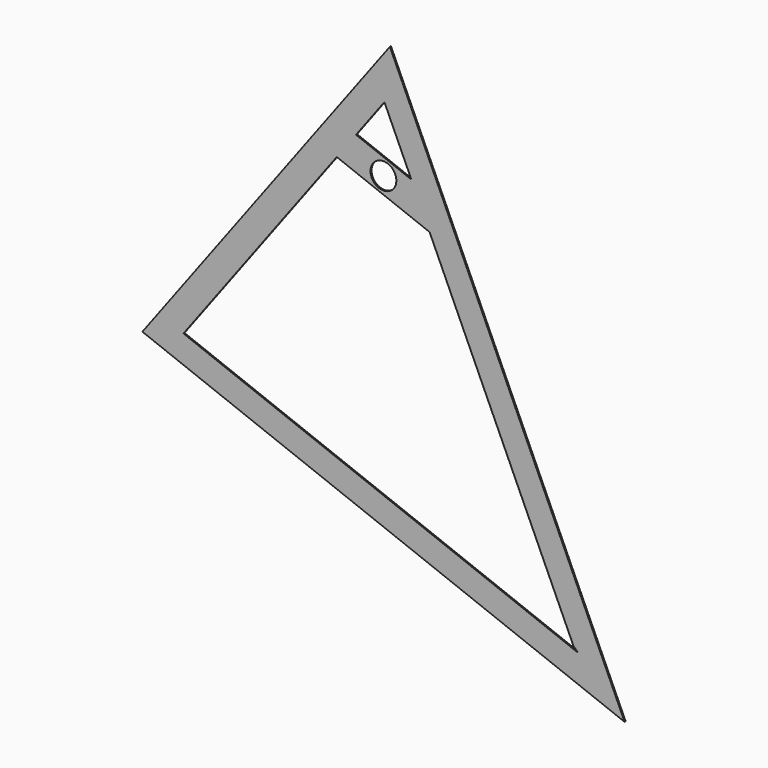
from build123d import *

# Parameters (mm, degrees)
F1_DEPTH = 25


# Not quite as in the source:
# - a feature names something its author has since deleted; it is built from what else it names


with BuildPart() as f1:
    # F0 (on Front) → F1 (new body)
    with BuildSketch(Plane.XZ):
        Polygon((5704.0546409884, -457.5102814203), (3652.3110417295, -3204.934271635), (4012.161188687, -3558.6994219099), (5018.0213600066, -2211.7843558738), (5390.744898264, -1712.6822306881), (5939.6636085267, -977.6428067571), align=None)
        Polygon((6045.7178843911, 0), (5704.0546409884, -457.5102814203), (5939.6636085267, -977.6428067571), (6281.3268519294, -520.1325253368), align=None)
        Polygon((6281.3268519294, -520.1325253368), (5939.6636085267, -977.6428067571), (6460.143900134, -2126.6598891299), (6813.5573514414, -2906.8586771351), (7811.482530577, -5109.8874877281), (8315.1269391623, -5009.9683174769), align=None)
        Polygon((9684.9106265398, -9135.5237592666), (10290.0247845106, -9369.7709782828), (8315.1269391623, -5009.9683174769), (7811.482530577, -5109.8874877281), (9594.9480898004, -9047.0824716979), align=None)
        Polygon((9684.9106265398, -9135.5237592666), (10584.5359939335, -10019.9366349539), (10290.0247845106, -9369.7709782828), align=None)
        Polygon((9624.3992107427, -9112.099037365), (9918.9104201656, -9762.264694036), (10584.5359939335, -10019.9366349539), (9684.9106265398, -9135.5237592666), align=None)
        Polygon((1991.4778842829, -6264.5315683592), (1258.904199068, -6409.8685432701), (1742.9955254446, -6597.266318483), align=None)
        Polygon((1569.5071476159, -5993.9501056153), (1258.904199068, -6409.8685432701), (1991.4778842829, -6264.5315683592), (2053.5984739925, -6181.3478808282), align=None)
        Polygon((3652.3110417295, -3204.934271635), (1569.5071476159, -5993.9501056153), (2053.5984739925, -6181.3478808282), (4012.161188687, -3558.6994219099), align=None)
        Polygon((1991.4778842829, -6264.5315683592), (1742.9955254446, -6597.266318483), (9918.9104201656, -9762.264694036), (9624.3992107427, -9112.099037365), (2174.6213055867, -6228.1973246315), align=None)
        Polygon((2053.5984739925, -6181.3478808282), (1991.4778842829, -6264.5315683592), (2174.6213055866, -6228.1973246315), align=None)
        with BuildLine():
            Line((5390.744898264, -1712.6822306881), (5018.0213600066, -2211.7843558738))
            Line((5018.0213600066, -2211.7843558738), (5915.789355724, -2559.3215165045))
            Line((5915.789355724, -2559.3215165045), (5916.8437449333, -2489.467813527))
            ThreePointArc((5916.8437449333, -2489.467813527), (5670.6453521413, -2235.7231556785), (5924.3900099897, -1989.5247628865))
            Line((5924.3900099897, -1989.5247628865), (5925.444399199, -1919.671059909))
            Line((5925.444399199, -1919.671059909), (5390.744898264, -1712.6822306881))
        make_face()
        with BuildLine():
            Line((6813.5573514414, -2906.8586771351), (6460.143900134, -2126.6598891299))
            Line((6460.143900134, -2126.6598891299), (5925.444399199, -1919.671059909))
            Line((5925.444399199, -1919.671059909), (5924.3900099897, -1989.5247628865))
            ThreePointArc((5924.3900099897, -1989.5247628865), (6098.7225808122, -2064.058668427), (6170.6168774615, -2239.4962882067))
            ThreePointArc((6170.6168774615, -2239.4962882067), (6096.0544972412, -2417.6019915574), (5916.8437449333, -2489.467813527))
            Line((5916.8437449333, -2489.467813527), (5915.789355724, -2559.3215165045))
            Line((5915.789355724, -2559.3215165045), (6813.5573514414, -2906.8586771351))
        make_face()
    extrude(amount=F1_DEPTH)


solid = f1.part
